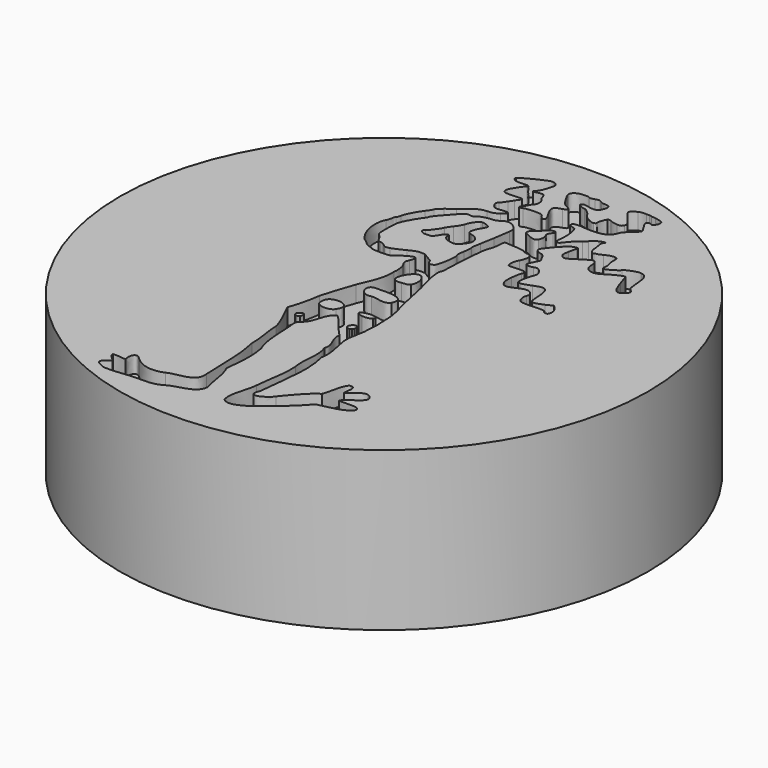
from build123d import *

# Parameters (mm, degrees)
F0_R     = 80
F1_DEPTH = 48
F3_DEPTH = 5


# Not quite as in the source:
# - ends of sketch curves that miss each other by under 0.0002 mm in the source are joined


with BuildPart() as f1:
    # F0 (on Top) → F1 (new body)
    with BuildSketch(Plane.XY):
        Circle(F0_R)
    extrude(amount=F1_DEPTH)

    # F2 (on face) → F3 (cut)
    with BuildSketch(Plane.XY.offset(48)):
        with BuildLine():
            add(Edge.make_bspline(
                [(24.522725, 70.595034), (24.233063, 70.702186), (24.086779, 70.724752), (23.891583, 70.722918)],
                knots=[0, 0, 0, 0, 1, 1, 1, 1], degree=3))
            add(Edge.make_bspline(
                [(23.891583, 70.722918), (23.696395, 70.720937), (23.451897, 70.694859), (22.966103, 70.705838)],
                knots=[0, 0, 0, 0, 1, 1, 1, 1], degree=3))
            add(Edge.make_bspline(
                [(22.966103, 70.705838), (22.184409, 70.723505), (21.250285, 70.779224), (20.571622, 70.377314)],
                knots=[0, 0, 0, 0, 1, 1, 1, 1], degree=3))
            add(Edge.make_bspline(
                [(20.571622, 70.377314), (19.890033, 69.973671), (18.8612, 69.219207), (18.8612, 68.802492)],
                knots=[0, 0, 0, 0, 1, 1, 1, 1], degree=3))
            add(Edge.make_bspline(
                [(18.8612, 68.802492), (18.8612, 68.689275), (19.337049, 68.113525), (19.831339, 67.453667)],
                knots=[0, 0, 0, 0, 1, 1, 1, 1], degree=3))
            add(Edge.make_bspline(
                [(19.831339, 67.453667), (21.496927, 65.230168), (22.01242, 64.899948), (22.413232, 64.067551)],
                knots=[0, 0, 0, 0, 1, 1, 1, 1], degree=3))
            add(Edge.make_bspline(
                [(22.413232, 64.067551), (22.937084, 63.513009), (22.843567, 63.926617), (22.422602, 62.96512)],
                knots=[0, 0, 0, 0, 1, 1, 1, 1], degree=3))
            add(Edge.make_bspline(
                [(22.422602, 62.96512), (22.164591, 62.288128), (21.88761, 62.167018), (20.751869, 62.235863)],
                knots=[0, 0, 0, 0, 1, 1, 1, 1], degree=3))
            add(Edge.make_bspline(
                [(20.751869, 62.235863), (20.002978, 62.281262), (19.029935, 62.508202), (18.589451, 62.740226)],
                knots=[0, 0, 0, 0, 1, 1, 1, 1], degree=3))
            add(Edge.make_bspline(
                [(18.589451, 62.740226), (18.100083, 62.997999), (17.672664, 63.03436), (17.490881, 62.833932)],
                knots=[0, 0, 0, 0, 1, 1, 1, 1], degree=3))
            add(Edge.make_bspline(
                [(17.490881, 62.833932), (17.038191, 62.334819), (16.376702, 60.170166), (16.577517, 59.845244)],
                knots=[0, 0, 0, 0, 1, 1, 1, 1], degree=3))
            add(Edge.make_bspline(
                [(16.577517, 59.845244), (16.675025, 59.687473), (16.42429, 59.453686), (16.020238, 59.325447)],
                knots=[0, 0, 0, 0, 1, 1, 1, 1], degree=3))
            add(Edge.make_bspline(
                [(16.020238, 59.325447), (15.219529, 59.071311), (12.594199, 60.644373), (12.228428, 61.597556)],
                knots=[0, 0, 0, 0, 1, 1, 1, 1], degree=3))
            add(Edge.make_bspline(
                [(12.228428, 61.597556), (11.952922, 62.315509), (10.32579, 63.715941), (9.751267, 63.729657)],
                knots=[0, 0, 0, 0, 1, 1, 1, 1], degree=3))
            add(Edge.make_bspline(
                [(9.751267, 63.729657), (9.494504, 63.735781), (7.426648, 64.17), (7.647828, 64.937921)],
                knots=[0, 0, 0, 0, 1, 1, 1, 1], degree=3))
            add(Edge.make_bspline(
                [(7.647828, 64.937921), (8.277054, 65.725744), (9.846808, 64.956576), (10.980478, 64.886105)],
                knots=[0, 0, 0, 0, 1, 1, 1, 1], degree=3))
            add(Edge.make_bspline(
                [(10.980478, 64.886105), (12.577906, 64.786825), (13.067226, 65.165762), (13.559613, 66.882607)],
                knots=[0, 0, 0, 0, 1, 1, 1, 1], degree=3))
            add(Edge.make_bspline(
                [(13.559613, 66.882607), (13.916173, 68.125864), (13.360638, 68.640806), (11.806198, 68.507592)],
                knots=[0, 0, 0, 0, 1, 1, 1, 1], degree=3))
            add(Edge.make_bspline(
                [(11.806198, 68.507592), (11.321405, 68.466043), (10.853308, 68.801899), (10.525724, 68.977227)],
                knots=[0, 0, 0, 0, 1, 1, 1, 1], degree=3))
            add(Edge.make_bspline(
                [(10.525724, 68.977227), (9.877545, 69.324143), (9.924196, 69.461782), (8.597574, 69.064318)],
                knots=[0, 0, 0, 0, 1, 1, 1, 1], degree=3))
            add(Edge.make_bspline(
                [(8.597574, 69.064318), (7.506288, 68.73736), (7.030529, 68.71743), (6.937864, 68.995416)],
                knots=[0, 0, 0, 0, 1, 1, 1, 1], degree=3))
            add(Edge.make_bspline(
                [(6.937864, 68.995416), (6.866423, 69.209738), (5.719491, 69.108415), (4.974436, 69.108415)],
                knots=[0, 0, 0, 0, 1, 1, 1, 1], degree=3))
            add(Edge.make_bspline(
                [(4.974436, 69.108415), (3.344859, 69.108415), (1.845701, 67.945318), (2.159379, 66.98734)],
                knots=[0, 0, 0, 0, 1, 1, 1, 1], degree=3))
            add(Edge.make_bspline(
                [(2.159379, 66.98734), (2.644291, 65.506427), (3.555651, 64.36065), (3.708294, 64.093459)],
                knots=[0, 0, 0, 0, 1, 1, 1, 1], degree=3))
            Line((3.708294, 64.093459), (4.061072, 63.476097))
            add(Edge.make_bspline(
                [(4.061072, 63.476097), (4.241169, 63.16085), (4.670435, 62.567618), (5.51683, 62.152077)],
                knots=[0, 0, 0, 0, 1, 1, 1, 1], degree=3))
            add(Edge.make_bspline(
                [(5.51683, 62.152077), (7.271411, 61.290653), (7.334279, 60.85184), (5.768186, 60.389292)],
                knots=[0, 0, 0, 0, 1, 1, 1, 1], degree=3))
            add(Edge.make_bspline(
                [(5.768186, 60.389292), (3.30002, 59.660317), (3.118873, 58.929393), (4.750089, 56.278327)],
                knots=[0, 0, 0, 0, 1, 1, 1, 1], degree=3))
            add(Edge.make_bspline(
                [(4.750089, 56.278327), (5.332172, 55.332321), (5.808422, 54.322457), (5.808422, 54.03433)],
                knots=[0, 0, 0, 0, 1, 1, 1, 1], degree=3))
            add(Edge.make_bspline(
                [(5.808422, 54.03433), (5.808422, 53.210239), (4.889352, 53.42155), (4.253446, 54.39207)],
                knots=[0, 0, 0, 0, 1, 1, 1, 1], degree=3))
            add(Edge.make_bspline(
                [(4.253446, 54.39207), (3.73622, 55.181454), (3.437231, 55.274014), (1.406969, 55.274014)],
                knots=[0, 0, 0, 0, 1, 1, 1, 1], degree=3))
            add(Edge.make_bspline(
                [(1.406969, 55.274014), (0.159392, 55.274014), (-1.266395, 55.089458), (-1.761416, 54.863911)],
                knots=[0, 0, 0, 0, 1, 1, 1, 1], degree=3))
            add(Edge.make_bspline(
                [(-1.761416, 54.863911), (-2.993516, 54.302529), (-3.294449, 54.750966), (-2.356176, 55.749714)],
                knots=[0, 0, 0, 0, 1, 1, 1, 1], degree=3))
            add(Edge.make_bspline(
                [(-2.356176, 55.749714), (-1.929724, 56.203648), (-1.687482, 57.017572), (-1.423522, 57.390681)],
                knots=[0, 0, 0, 0, 1, 1, 1, 1], degree=3))
            add(Edge.make_bspline(
                [(-1.423522, 57.390681), (-1.03471, 57.940266), (-0.466679, 58.411795), (-0.481495, 59.042121)],
                knots=[0, 0, 0, 0, 1, 1, 1, 1], degree=3))
            Line((-0.481495, 59.042121), (-1.001298, 60.953186))
            add(Edge.make_bspline(
                [(-1.001298, 60.953186), (-1.99067, 61.768707), (-1.593124, 62.769955), (-2.273976, 63.235297)],
                knots=[0, 0, 0, 0, 1, 1, 1, 1], degree=3))
            add(Edge.make_bspline(
                [(-2.273976, 63.235297), (-3.104235, 63.80275), (-5.087721, 62.734017), (-5.282036, 62.999297)],
                knots=[0, 0, 0, 0, 1, 1, 1, 1], degree=3))
            add(Edge.make_bspline(
                [(-5.282036, 62.999297), (-5.39946, 63.189292), (-5.293607, 63.473543), (-5.046668, 63.630989)],
                knots=[0, 0, 0, 0, 1, 1, 1, 1], degree=3))
            add(Edge.make_bspline(
                [(-5.046668, 63.630989), (-4.481129, 63.991582), (-3.871625, 65.249317), (-3.319711, 67.195699)],
                knots=[0, 0, 0, 0, 1, 1, 1, 1], degree=3))
            add(Edge.make_bspline(
                [(-3.319711, 67.195699), (-2.952041, 68.492326), (-2.970916, 68.790489), (-3.448695, 69.268268)],
                knots=[0, 0, 0, 0, 1, 1, 1, 1], degree=3))
            add(Edge.make_bspline(
                [(-3.448695, 69.268268), (-3.755629, 69.575205), (-4.378445, 69.826097), (-4.832795, 69.826097)],
                knots=[0, 0, 0, 0, 1, 1, 1, 1], degree=3))
            add(Edge.make_bspline(
                [(-4.832795, 69.826097), (-5.867523, 69.826097), (-12.562215, 66.553353), (-12.801164, 65.93066)],
                knots=[0, 0, 0, 0, 1, 1, 1, 1], degree=3))
            add(Edge.make_bspline(
                [(-12.801164, 65.93066), (-13.103503, 65.142783), (-11.77094, 64.413888), (-10.33117, 64.579631)],
                knots=[0, 0, 0, 0, 1, 1, 1, 1], degree=3))
            add(Edge.make_bspline(
                [(-10.33117, 64.579631), (-9.158629, 64.71461), (-7.35364, 64.903716), (-8.086619, 64.186614)],
                knots=[0, 0, 0, 0, 1, 1, 1, 1], degree=3))
            add(Edge.make_bspline(
                [(-8.086619, 64.186614), (-8.451558, 63.829584), (-10.772142, 60.580706), (-10.772142, 59.695313)],
                knots=[0, 0, 0, 0, 1, 1, 1, 1], degree=3))
            add(Edge.make_bspline(
                [(-10.772142, 59.695313), (-10.772142, 58.627779), (-10.244513, 58.293024), (-8.72217, 58.395547)],
                knots=[0, 0, 0, 0, 1, 1, 1, 1], degree=3))
            add(Edge.make_bspline(
                [(-8.72217, 58.395547), (-7.82656, 58.455864), (-6.579872, 58.530695), (-5.651349, 58.549886)],
                knots=[0, 0, 0, 0, 1, 1, 1, 1], degree=3))
            add(Edge.make_bspline(
                [(-5.651349, 58.549886), (-3.885942, 58.586366), (-5.648809, 57.191723), (-5.842072, 56.658117)],
                knots=[0, 0, 0, 0, 1, 1, 1, 1], degree=3))
            Line((-5.842072, 56.658117), (-6.67165, 55.343466))
            add(Edge.make_bspline(
                [(-6.67165, 55.343466), (-7.128023, 54.620523), (-7.751509, 53.821326), (-8.057407, 53.567453)],
                knots=[0, 0, 0, 0, 1, 1, 1, 1], degree=3))
            add(Edge.make_bspline(
                [(-8.057407, 53.567453), (-8.656912, 53.069906), (-8.521332, 52.301858), (-7.656121, 51.295341)],
                knots=[0, 0, 0, 0, 1, 1, 1, 1], degree=3))
            add(Edge.make_bspline(
                [(-7.656121, 51.295341), (-7.204923, 50.77045), (-6.780399, 50.705353), (-5.063754, 50.89957)],
                knots=[0, 0, 0, 0, 1, 1, 1, 1], degree=3))
            add(Edge.make_bspline(
                [(-5.063754, 50.89957), (-2.627062, 51.17525), (-2.439217, 50.807322), (-4.294809, 49.391995)],
                knots=[0, 0, 0, 0, 1, 1, 1, 1], degree=3))
            add(Edge.make_bspline(
                [(-4.294809, 49.391995), (-5.284181, 48.637364), (-6.002764, 48.400218), (-7.426265, 48.359019)],
                knots=[0, 0, 0, 0, 1, 1, 1, 1], degree=3))
            add(Edge.make_bspline(
                [(-7.426265, 48.359019), (-9.266164, 48.305767), (-10.477911, 47.639505), (-13.85674, 44.821869)],
                knots=[0, 0, 0, 0, 1, 1, 1, 1], degree=3))
            add(Edge.make_bspline(
                [(-13.85674, 44.821869), (-14.29202, 44.458883), (-15.363584, 43.606643), (-16.23799, 42.928446)],
                knots=[0, 0, 0, 0, 1, 1, 1, 1], degree=3))
            add(Edge.make_bspline(
                [(-16.23799, 42.928446), (-17.112397, 42.250252), (-17.827697, 41.518997), (-17.827697, 41.303464)],
                knots=[0, 0, 0, 0, 1, 1, 1, 1], degree=3))
            add(Edge.make_bspline(
                [(-17.827697, 41.303464), (-17.827697, 41.087928), (-18.359957, 40.214052), (-19.010604, 39.361532)],
                knots=[0, 0, 0, 0, 1, 1, 1, 1], degree=3))
            add(Edge.make_bspline(
                [(-19.010604, 39.361532), (-20.451382, 37.473734), (-21.538646, 35.376204), (-21.868657, 33.847175)],
                knots=[0, 0, 0, 0, 1, 1, 1, 1], degree=3))
            add(Edge.make_bspline(
                [(-21.868657, 33.847175), (-22.004279, 33.218807), (-22.262266, 32.614005), (-22.441367, 32.503312)],
                knots=[0, 0, 0, 0, 1, 1, 1, 1], degree=3))
            add(Edge.make_bspline(
                [(-22.441367, 32.503312), (-22.620468, 32.392622), (-22.766586, 31.986114), (-22.766586, 31.599871)],
                knots=[0, 0, 0, 0, 1, 1, 1, 1], degree=3))
            add(Edge.make_bspline(
                [(-22.766586, 31.599871), (-22.766586, 31.21363), (-23.001545, 30.443423), (-23.288587, 29.888345)],
                knots=[0, 0, 0, 0, 1, 1, 1, 1], degree=3))
            add(Edge.make_bspline(
                [(-23.288587, 29.888345), (-24.543423, 27.461756), (-24.119368, 23.492182), (-22.297502, 20.613597)],
                knots=[0, 0, 0, 0, 1, 1, 1, 1], degree=3))
            add(Edge.make_bspline(
                [(-22.297502, 20.613597), (-21.714196, 19.691967), (-21.13351, 18.937903), (-21.007106, 18.937903)],
                knots=[0, 0, 0, 0, 1, 1, 1, 1], degree=3))
            add(Edge.make_bspline(
                [(-21.007106, 18.937903), (-20.880701, 18.937903), (-20.243562, 18.461653), (-19.591586, 17.87957)],
                knots=[0, 0, 0, 0, 1, 1, 1, 1], degree=3))
            add(Edge.make_bspline(
                [(-19.591586, 17.87957), (-18.939611, 17.297486), (-18.126912, 16.821236), (-17.785254, 16.821236)],
                knots=[0, 0, 0, 0, 1, 1, 1, 1], degree=3))
            add(Edge.make_bspline(
                [(-17.785254, 16.821236), (-17.443596, 16.821236), (-17.065669, 16.662486), (-16.945753, 16.468459)],
                knots=[0, 0, 0, 0, 1, 1, 1, 1], degree=3))
            add(Edge.make_bspline(
                [(-16.945753, 16.468459), (-16.648025, 15.986728), (-11.229864, 16.013584), (-10.930339, 16.498224)],
                knots=[0, 0, 0, 0, 1, 1, 1, 1], degree=3))
            add(Edge.make_bspline(
                [(-10.930339, 16.498224), (-10.800474, 16.708353), (-9.846244, 17.422728), (-8.809814, 18.085724)],
                knots=[0, 0, 0, 0, 1, 1, 1, 1], degree=3))
            add(Edge.make_bspline(
                [(-8.809814, 18.085724), (-5.96062, 19.90833), (-5.06882, 19.657067), (-6.049878, 17.309063)],
                knots=[0, 0, 0, 0, 1, 1, 1, 1], degree=3))
            add(Edge.make_bspline(
                [(-6.049878, 17.309063), (-6.574586, 16.053267), (-6.570516, 15.87637), (-5.992003, 14.802134)],
                knots=[0, 0, 0, 0, 1, 1, 1, 1], degree=3))
            Line((-5.992003, 14.802134), (-5.388973, 13.682618))
            add(Edge.make_bspline(
                [(-5.388973, 13.682618), (-5.278994, 12.380882), (-4.98303, 11.387617), (-5.299125, 10.435408)],
                knots=[0, 0, 0, 0, 1, 1, 1, 1], degree=3))
            add(Edge.make_bspline(
                [(-5.299125, 10.435408), (-4.924624, 6.564533), (-6.784054, 3.047559), (-8.216707, -0.421328)],
                knots=[0, 0, 0, 0, 1, 1, 1, 1], degree=3))
            add(Edge.make_bspline(
                [(-8.216707, -0.421328), (-9.516716, -3.60075), (-10.262812, -7.024907), (-11.352018, -10.214769)],
                knots=[0, 0, 0, 0, 1, 1, 1, 1], degree=3))
            add(Edge.make_bspline(
                [(-11.352018, -10.214769), (-11.76474, -13.396102), (-12.493974, -16.532977), (-13.600976, -19.556215)],
                knots=[0, 0, 0, 0, 1, 1, 1, 1], degree=3))
            add(Edge.make_bspline(
                [(-13.600976, -19.556215), (-12.288014, -22.651919), (-10.395127, -25.54803), (-9.642149, -28.840886)],
                knots=[0, 0, 0, 0, 1, 1, 1, 1], degree=3))
            add(Edge.make_bspline(
                [(-9.642149, -28.840886), (-9.594586, -32.330778), (-8.556401, -35.691054), (-8.657129, -39.19326)],
                knots=[0, 0, 0, 0, 1, 1, 1, 1], degree=3))
            add(Edge.make_bspline(
                [(-8.657129, -39.19326), (-7.144872, -45.432631), (-7.605439, -51.929971), (-7.175462, -58.301688)],
                knots=[0, 0, 0, 0, 1, 1, 1, 1], degree=3))
            add(Edge.make_bspline(
                [(-7.175462, -58.301688), (-6.548257, -63.167792), (-12.406347, -62.239501), (-15.176902, -63.733365)],
                knots=[0, 0, 0, 0, 1, 1, 1, 1], degree=3))
            add(Edge.make_bspline(
                [(-15.176902, -63.733365), (-18.35449, -65.081752), (-21.9356, -64.681172), (-24.805532, -61.775448)],
                knots=[0, 0, 0, 0, 1, 1, 1, 1], degree=3))
            add(Edge.make_bspline(
                [(-24.805532, -61.775448), (-26.688817, -59.868676), (-27.554608, -62.666003), (-26.80975, -64.276313)],
                knots=[0, 0, 0, 0, 1, 1, 1, 1], degree=3))
            add(Edge.make_bspline(
                [(-26.80975, -64.276313), (-27.921759, -64.34338), (-29.646639, -63.821187), (-30.850709, -64.100474)],
                knots=[0, 0, 0, 0, 1, 1, 1, 1], degree=3))
            add(Edge.make_bspline(
                [(-30.850709, -64.100474), (-30.948059, -65.198186), (-29.302621, -65.920497), (-28.85531, -66.779381)],
                knots=[0, 0, 0, 0, 1, 1, 1, 1], degree=3))
            add(Edge.make_bspline(
                [(-28.85531, -66.779381), (-29.513899, -67.358645), (-31.134712, -68.204657), (-31.027648, -68.991958)],
                knots=[0, 0, 0, 0, 1, 1, 1, 1], degree=3))
            add(Edge.make_bspline(
                [(-31.027648, -68.991958), (-30.9415, -69.625482), (-29.687355, -70.078505), (-28.880115, -70.481894)],
                knots=[0, 0, 0, 0, 1, 1, 1, 1], degree=3))
            add(Edge.make_bspline(
                [(-28.880115, -70.481894), (-27.886806, -70.978264), (-24.254227, -70.618213), (-20.843947, -70.234396)],
                knots=[0, 0, 0, 0, 1, 1, 1, 1], degree=3))
            add(Edge.make_bspline(
                [(-20.843947, -70.234396), (-17.203879, -69.82472), (-14.587414, -70.820267), (-11.188309, -68.767061)],
                knots=[0, 0, 0, 0, 1, 1, 1, 1], degree=3))
            add(Edge.make_bspline(
                [(-11.188309, -68.767061), (-8.339423, -67.046211), (-3.293405, -67.463691), (-2.78448, -63.458859)],
                knots=[0, 0, 0, 0, 1, 1, 1, 1], degree=3))
            add(Edge.make_bspline(
                [(-2.78448, -63.458859), (-3.80083, -60.019916), (-3.686905, -56.22129), (-5.34653, -52.992936)],
                knots=[0, 0, 0, 0, 1, 1, 1, 1], degree=3))
            add(Edge.make_bspline(
                [(-5.34653, -52.992936), (-4.769221, -48.662913), (-4.445165, -44.226047), (-5.272116, -39.898265)],
                knots=[0, 0, 0, 0, 1, 1, 1, 1], degree=3))
            add(Edge.make_bspline(
                [(-5.272116, -39.898265), (-7.076828, -35.924105), (-6.637115, -31.423476), (-7.08396, -27.18283)],
                knots=[0, 0, 0, 0, 1, 1, 1, 1], degree=3))
            add(Edge.make_bspline(
                [(-7.08396, -27.18283), (-7.080348, -25.874589), (-7.812994, -24.338671), (-6.495812, -23.43677)],
                knots=[0, 0, 0, 0, 1, 1, 1, 1], degree=3))
            add(Edge.make_bspline(
                [(-6.495812, -23.43677), (-3.657511, -21.438298), (-4.723445, -17.065558), (-1.698034, -15.503131)],
                knots=[0, 0, 0, 0, 1, 1, 1, 1], degree=3))
            add(Edge.make_bspline(
                [(-1.698034, -15.503131), (0.752634, -17.577222), (2.513396, -20.758016), (4.987655, -23.098324)],
                knots=[0, 0, 0, 0, 1, 1, 1, 1], degree=3))
            add(Edge.make_bspline(
                [(4.987655, -23.098324), (4.468572, -25.888734), (7.265903, -27.84126), (6.248836, -30.426181)],
                knots=[0, 0, 0, 0, 1, 1, 1, 1], degree=3))
            add(Edge.make_bspline(
                [(6.248836, -30.426181), (7.792834, -34.182745), (6.084712, -38.118975), (6.863993, -42.052413)],
                knots=[0, 0, 0, 0, 1, 1, 1, 1], degree=3))
            add(Edge.make_bspline(
                [(6.863993, -42.052413), (7.267404, -46.592401), (5.98027, -50.972433), (5.675021, -55.459623)],
                knots=[0, 0, 0, 0, 1, 1, 1, 1], degree=3))
            add(Edge.make_bspline(
                [(5.675021, -55.459623), (5.45009, -58.853489), (3.239842, -62.464308), (4.27383, -65.71829)],
                knots=[0, 0, 0, 0, 1, 1, 1, 1], degree=3))
            add(Edge.make_bspline(
                [(4.27383, -65.71829), (6.321254, -67.698903), (9.067304, -65.697152), (11.100634, -64.674288)],
                knots=[0, 0, 0, 0, 1, 1, 1, 1], degree=3))
            add(Edge.make_bspline(
                [(11.100634, -64.674288), (14.302829, -62.398968), (20.279166, -57.238122), (22.590716, -54.275613)],
                knots=[0, 0, 0, 0, 1, 1, 1, 1], degree=3))
            add(Edge.make_bspline(
                [(22.590716, -54.275613), (29.35799, -52.498403), (26.515086, -53.637283), (29.357984, -52.498494)],
                knots=[0, 0, 0, 0, 1, 1, 1, 1], degree=3))
            add(Edge.make_bspline(
                [(29.357984, -52.498494), (31.767933, -51.533133), (32.611854, -50.238955), (31.417876, -49.594142)],
                knots=[0, 0, 0, 0, 1, 1, 1, 1], degree=3))
            add(Edge.make_bspline(
                [(31.417876, -49.594142), (30.252369, -48.964704), (27.262572, -49.627252), (25.780047, -49.225379)],
                knots=[0, 0, 0, 0, 1, 1, 1, 1], degree=3))
            add(Edge.make_bspline(
                [(25.780047, -49.225379), (27.399413, -46.878346), (32.183263, -45.657675), (30.386001, -43.392419)],
                knots=[0, 0, 0, 0, 1, 1, 1, 1], degree=3))
            add(Edge.make_bspline(
                [(30.386001, -43.392419), (28.576624, -41.111891), (25.640124, -44.473697), (24.21239, -45.430811)],
                knots=[0, 0, 0, 0, 1, 1, 1, 1], degree=3))
            add(Edge.make_bspline(
                [(24.21239, -45.430811), (24.106323, -44.2573), (25.213703, -41.723009), (23.404859, -41.664358)],
                knots=[0, 0, 0, 0, 1, 1, 1, 1], degree=3))
            add(Edge.make_bspline(
                [(23.404859, -41.664358), (21.655973, -41.607651), (21.36426, -47.486179), (20.491688, -49.066076)],
                knots=[0, 0, 0, 0, 1, 1, 1, 1], degree=3))
            add(Edge.make_bspline(
                [(20.491688, -49.066076), (17.432701, -51.023665), (15.187742, -54.106751), (12.836961, -56.890027)],
                knots=[0, 0, 0, 0, 1, 1, 1, 1], degree=3))
            add(Edge.make_bspline(
                [(12.836961, -56.890027), (11.70214, -58.882414), (6.153837, -61.653105), (8.193525, -57.148548)],
                knots=[0, 0, 0, 0, 1, 1, 1, 1], degree=3))
            add(Edge.make_bspline(
                [(8.193525, -57.148548), (8.861993, -52.678819), (9.028414, -48.153256), (9.525811, -43.663617)],
                knots=[0, 0, 0, 0, 1, 1, 1, 1], degree=3))
            add(Edge.make_bspline(
                [(9.525811, -43.663617), (9.752074, -40.723739), (9.420867, -37.419326), (8.7271, -34.521711)],
                knots=[0, 0, 0, 0, 1, 1, 1, 1], degree=3))
            add(Edge.make_bspline(
                [(8.7271, -34.521711), (9.575747, -30.47423), (7.287817, -26.702595), (7.642858, -22.693182)],
                knots=[0, 0, 0, 0, 1, 1, 1, 1], degree=3))
            add(Edge.make_bspline(
                [(7.642858, -22.693182), (8.740491, -18.063412), (8.900751, -13.274402), (8.485667, -8.540729)],
                knots=[0, 0, 0, 0, 1, 1, 1, 1], degree=3))
            add(Edge.make_bspline(
                [(8.485667, -8.540729), (8.260499, -4.973321), (6.723406, -1.712308), (6.232851, 1.721244)],
                knots=[0, 0, 0, 0, 1, 1, 1, 1], degree=3))
            add(Edge.make_bspline(
                [(6.232851, 1.721244), (5.362816, 5.562302), (4.627458, 9.90049), (3.427164, 13.667733)],
                knots=[0, 0, 0, 0, 1, 1, 1, 1], degree=3))
            Line((3.427164, 13.667733), (3.198962, 15.384217))
            add(Edge.make_bspline(
                [(3.198962, 15.384217), (3.069015, 16.363805), (3.113561, 17.211451), (3.300937, 17.327252)],
                knots=[0, 0, 0, 0, 1, 1, 1, 1], degree=3))
            add(Edge.make_bspline(
                [(3.300937, 17.327252), (3.483747, 17.440237), (3.624779, 18.682608), (3.614026, 20.087738)],
                knots=[0, 0, 0, 0, 1, 1, 1, 1], degree=3))
            add(Edge.make_bspline(
                [(3.614026, 20.087738), (3.603273, 21.492872), (3.713052, 23.832695), (3.858216, 25.287903)],
                knots=[0, 0, 0, 0, 1, 1, 1, 1], degree=3))
            add(Edge.make_bspline(
                [(3.858216, 25.287903), (4.00338, 26.743111), (4.171017, 28.648111), (4.230837, 29.521236)],
                knots=[0, 0, 0, 0, 1, 1, 1, 1], degree=3))
            add(Edge.make_bspline(
                [(4.230837, 29.521236), (4.379094, 31.685215), (4.619705, 32.941304), (5.113885, 34.134356)],
                knots=[0, 0, 0, 0, 1, 1, 1, 1], degree=3))
            add(Edge.make_bspline(
                [(5.113885, 34.134356), (5.343478, 34.688649), (5.553629, 35.901578), (5.581315, 36.829798)],
                knots=[0, 0, 0, 0, 1, 1, 1, 1], degree=3))
            add(Edge.make_bspline(
                [(5.581315, 36.829798), (5.628342, 38.405787), (5.690391, 38.51149), (6.513969, 38.432733)],
                knots=[0, 0, 0, 0, 1, 1, 1, 1], degree=3))
            add(Edge.make_bspline(
                [(6.513969, 38.432733), (6.999039, 38.386347), (8.389627, 38.29806), (9.604083, 38.235951)],
                knots=[0, 0, 0, 0, 1, 1, 1, 1], degree=3))
            add(Edge.make_bspline(
                [(9.604083, 38.235951), (10.818533, 38.173842), (12.001222, 37.933979), (12.232277, 37.702926)],
                knots=[0, 0, 0, 0, 1, 1, 1, 1], degree=3))
            add(Edge.make_bspline(
                [(12.232277, 37.702926), (12.463327, 37.471874), (13.079531, 37.282347), (13.602048, 37.282347)],
                knots=[0, 0, 0, 0, 1, 1, 1, 1], degree=3))
            add(Edge.make_bspline(
                [(13.602048, 37.282347), (15.144847, 37.282347), (15.426578, 35.658912), (14.27508, 33.401792)],
                knots=[0, 0, 0, 0, 1, 1, 1, 1], degree=3))
            add(Edge.make_bspline(
                [(14.27508, 33.401792), (13.480334, 31.843965), (13.346372, 30.010452), (14.010497, 29.780308)],
                knots=[0, 0, 0, 0, 1, 1, 1, 1], degree=3))
            add(Edge.make_bspline(
                [(14.010497, 29.780308), (14.253033, 29.696254), (15.421701, 29.70288), (16.607825, 29.795181)],
                knots=[0, 0, 0, 0, 1, 1, 1, 1], degree=3))
            add(Edge.make_bspline(
                [(16.607825, 29.795181), (18.934355, 29.976246), (19.499048, 29.65591), (18.882691, 28.504234)],
                knots=[0, 0, 0, 0, 1, 1, 1, 1], degree=3))
            add(Edge.make_bspline(
                [(18.882691, 28.504234), (18.682765, 28.130671), (18.417386, 26.724276), (18.292339, 25.378846)],
                knots=[0, 0, 0, 0, 1, 1, 1, 1], degree=3))
            add(Edge.make_bspline(
                [(18.292339, 25.378846), (18.106614, 23.380498), (18.17735, 22.760733), (18.679844, 21.993833)],
                knots=[0, 0, 0, 0, 1, 1, 1, 1], degree=3))
            add(Edge.make_bspline(
                [(18.679844, 21.993833), (19.447793, 20.821804), (20.164288, 20.816182), (22.590716, 21.964067)],
                knots=[0, 0, 0, 0, 1, 1, 1, 1], degree=3))
            add(Edge.make_bspline(
                [(22.590716, 21.964067), (23.997089, 22.629367), (24.801772, 22.80989), (25.590981, 22.636549)],
                knots=[0, 0, 0, 0, 1, 1, 1, 1], degree=3))
            add(Edge.make_bspline(
                [(25.590981, 22.636549), (26.760716, 22.379637), (27.434123, 21.241728), (26.956891, 20.328612)],
                knots=[0, 0, 0, 0, 1, 1, 1, 1], degree=3))
            add(Edge.make_bspline(
                [(26.956891, 20.328612), (26.508209, 19.470123), (26.824927, 17.803401), (27.535667, 17.283697)],
                knots=[0, 0, 0, 0, 1, 1, 1, 1], degree=3))
            add(Edge.make_bspline(
                [(27.535667, 17.283697), (28.013681, 16.934159), (29.060954, 16.860626), (31.594816, 16.998167)],
                knots=[0, 0, 0, 0, 1, 1, 1, 1], degree=3))
            add(Edge.make_bspline(
                [(31.594816, 16.998167), (34.435278, 17.152354), (35.044274, 17.09379), (35.214649, 16.6498)],
                knots=[0, 0, 0, 0, 1, 1, 1, 1], degree=3))
            add(Edge.make_bspline(
                [(35.214649, 16.6498), (35.327306, 16.356222), (35.74213, 16.115672), (36.136279, 16.115672)],
                knots=[0, 0, 0, 0, 1, 1, 1, 1], degree=3))
            add(Edge.make_bspline(
                [(36.136279, 16.115672), (37.246567, 16.115672), (37.141766, 18.543212), (35.984695, 19.630222)],
                knots=[0, 0, 0, 0, 1, 1, 1, 1], degree=3))
            Line((35.984695, 19.630222), (33.215389, 19.51557))
            add(Edge.make_bspline(
                [(33.215389, 19.51557), (31.181261, 18.520364), (29.988206, 18.34358), (29.595009, 18.979788)],
                knots=[0, 0, 0, 0, 1, 1, 1, 1], degree=3))
            add(Edge.make_bspline(
                [(29.595009, 18.979788), (29.460837, 19.196876), (29.312281, 20.347812), (29.264828, 21.537426)],
                knots=[0, 0, 0, 0, 1, 1, 1, 1], degree=3))
            add(Edge.make_bspline(
                [(29.264828, 21.537426), (29.087788, 25.975605), (28.18101, 26.739282), (24.787858, 25.307738)],
                knots=[0, 0, 0, 0, 1, 1, 1, 1], degree=3))
            add(Edge.make_bspline(
                [(24.787858, 25.307738), (23.504075, 24.766119), (22.085027, 24.34175), (21.634358, 24.36461)],
                knots=[0, 0, 0, 0, 1, 1, 1, 1], degree=3))
            add(Edge.make_bspline(
                [(21.634358, 24.36461), (20.88639, 24.402569), (20.825142, 24.544346), (20.929353, 25.99345)],
                knots=[0, 0, 0, 0, 1, 1, 1, 1], degree=3))
            add(Edge.make_bspline(
                [(20.929353, 25.99345), (20.992144, 26.866575), (21.266538, 28.116743), (21.539548, 28.771025)],
                knots=[0, 0, 0, 0, 1, 1, 1, 1], degree=3))
            add(Edge.make_bspline(
                [(21.539548, 28.771025), (22.238982, 30.447241), (22.163621, 31.111671), (21.148735, 32.20675)],
                knots=[0, 0, 0, 0, 1, 1, 1, 1], degree=3))
            add(Edge.make_bspline(
                [(21.148735, 32.20675), (20.331346, 33.088731), (20.161471, 33.133692), (19.000099, 32.777257)],
                knots=[0, 0, 0, 0, 1, 1, 1, 1], degree=3))
            add(Edge.make_bspline(
                [(19.000099, 32.777257), (17.725693, 32.386128), (16.744525, 32.516867), (16.744525, 33.077668)],
                knots=[0, 0, 0, 0, 1, 1, 1, 1], degree=3))
            add(Edge.make_bspline(
                [(16.744525, 33.077668), (16.744525, 33.245746), (17.085774, 34.085867), (17.502997, 34.944636)],
                knots=[0, 0, 0, 0, 1, 1, 1, 1], degree=3))
            Line((17.502997, 34.944636), (17.558671, 37.864422))
            add(Edge.make_bspline(
                [(17.558671, 37.864422), (17.090831, 38.768645), (16.57189, 39.263782), (16.006449, 39.344985)],
                knots=[0, 0, 0, 0, 1, 1, 1, 1], degree=3))
            add(Edge.make_bspline(
                [(16.006449, 39.344985), (14.960378, 39.495218), (14.27508, 40.028663), (14.27508, 40.692707)],
                knots=[0, 0, 0, 0, 1, 1, 1, 1], degree=3))
            add(Edge.make_bspline(
                [(14.27508, 40.692707), (14.27508, 41.403591), (17.678599, 45.413347), (19.115302, 46.395029)],
                knots=[0, 0, 0, 0, 1, 1, 1, 1], degree=3))
            add(Edge.make_bspline(
                [(19.115302, 46.395029), (20.24228, 47.165084), (21.627387, 47.220969), (21.168028, 46.477712)],
                knots=[0, 0, 0, 0, 1, 1, 1, 1], degree=3))
            add(Edge.make_bspline(
                [(21.168028, 46.477712), (21.054205, 46.293542), (20.795345, 45.245228), (20.59256, 44.148278)],
                knots=[0, 0, 0, 0, 1, 1, 1, 1], degree=3))
            add(Edge.make_bspline(
                [(20.59256, 44.148278), (20.272794, 42.418481), (20.304993, 42.064058), (20.836197, 41.477087)],
                knots=[0, 0, 0, 0, 1, 1, 1, 1], degree=3))
            add(Edge.make_bspline(
                [(20.836197, 41.477087), (21.599439, 40.633711), (22.077484, 40.780317), (25.040868, 42.767483)],
                knots=[0, 0, 0, 0, 1, 1, 1, 1], degree=3))
            add(Edge.make_bspline(
                [(25.040868, 42.767483), (26.328995, 43.631264), (27.576981, 44.337894), (27.814031, 44.337894)],
                knots=[0, 0, 0, 0, 1, 1, 1, 1], degree=3))
            add(Edge.make_bspline(
                [(27.814031, 44.337894), (28.604965, 44.337894), (29.091747, 43.504653), (29.091747, 42.150672)],
                knots=[0, 0, 0, 0, 1, 1, 1, 1], degree=3))
            add(Edge.make_bspline(
                [(29.091747, 42.150672), (29.091747, 39.526443), (31.565665, 38.563123), (34.036701, 40.225279)],
                knots=[0, 0, 0, 0, 1, 1, 1, 1], degree=3))
            add(Edge.make_bspline(
                [(34.036701, 40.225279), (36.349952, 41.7813), (38.986148, 42.945054), (39.142056, 42.478646)],
                knots=[0, 0, 0, 0, 1, 1, 1, 1], degree=3))
            add(Edge.make_bspline(
                [(39.142056, 42.478646), (39.221741, 42.240261), (39.703853, 40.774839), (40.213067, 39.222617)],
                knots=[0, 0, 0, 0, 1, 1, 1, 1], degree=3))
            add(Edge.make_bspline(
                [(40.213067, 39.222617), (41.539234, 35.180122), (42.444541, 34.409452), (44.172997, 35.851385)],
                knots=[0, 0, 0, 0, 1, 1, 1, 1], degree=3))
            add(Edge.make_bspline(
                [(44.172997, 35.851385), (45.153917, 36.669699), (45.183705, 37.399893), (44.262295, 38.033095)],
                knots=[0, 0, 0, 0, 1, 1, 1, 1], degree=3))
            add(Edge.make_bspline(
                [(44.262295, 38.033095), (43.684741, 38.42999), (43.516751, 39.07377), (43.327984, 41.610482)],
                knots=[0, 0, 0, 0, 1, 1, 1, 1], degree=3))
            add(Edge.make_bspline(
                [(43.327984, 41.610482), (43.069728, 45.080977), (42.507982, 46.110913), (40.763733, 46.314)],
                knots=[0, 0, 0, 0, 1, 1, 1, 1], degree=3))
            add(Edge.make_bspline(
                [(40.763733, 46.314), (39.712946, 46.436347), (36.717598, 45.32874), (36.30826, 44.666418)],
                knots=[0, 0, 0, 0, 1, 1, 1, 1], degree=3))
            add(Edge.make_bspline(
                [(36.30826, 44.666418), (35.980515, 44.136117), (33.524197, 42.645176), (32.760086, 42.51282)],
                knots=[0, 0, 0, 0, 1, 1, 1, 1], degree=3))
            add(Edge.make_bspline(
                [(32.760086, 42.51282), (32.205734, 42.416822), (32.113896, 42.586254), (32.206665, 43.536429)],
                knots=[0, 0, 0, 0, 1, 1, 1, 1], degree=3))
            add(Edge.make_bspline(
                [(32.206665, 43.536429), (32.267805, 44.162632), (32.187192, 44.877007), (32.027521, 45.123929)],
                knots=[0, 0, 0, 0, 1, 1, 1, 1], degree=3))
            add(Edge.make_bspline(
                [(32.027521, 45.123929), (31.86784, 45.37085), (31.73758, 46.286992), (31.73758, 47.160117)],
                knots=[0, 0, 0, 0, 1, 1, 1, 1], degree=3))
            add(Edge.make_bspline(
                [(31.73758, 47.160117), (31.73758, 48.638267), (31.66906, 48.755818), (30.745394, 48.861719)],
                knots=[0, 0, 0, 0, 1, 1, 1, 1], degree=3))
            add(Edge.make_bspline(
                [(30.745394, 48.861719), (30.170496, 48.927635), (29.020932, 48.59255), (28.011367, 48.064662)],
                knots=[0, 0, 0, 0, 1, 1, 1, 1], degree=3))
            add(Edge.make_bspline(
                [(28.011367, 48.064662), (27.05325, 47.563678), (26.269525, 47.254105), (26.269525, 47.376745)],
                knots=[0, 0, 0, 0, 1, 1, 1, 1], degree=3))
            add(Edge.make_bspline(
                [(26.269525, 47.376745), (26.269525, 47.499382), (26.061716, 47.427322), (25.808159, 47.216891)],
                knots=[0, 0, 0, 0, 1, 1, 1, 1], degree=3))
            add(Edge.make_bspline(
                [(25.808159, 47.216891), (25.456959, 46.925418), (25.207176, 47.071482), (24.759196, 47.829844)],
                knots=[0, 0, 0, 0, 1, 1, 1, 1], degree=3))
            add(Edge.make_bspline(
                [(24.759196, 47.829844), (24.43578, 48.377347), (24.252113, 48.90585), (24.350747, 49.004484)],
                knots=[0, 0, 0, 0, 1, 1, 1, 1], degree=3))
            add(Edge.make_bspline(
                [(24.350747, 49.004484), (24.449381, 49.103115), (24.374962, 49.874409), (24.185382, 50.718211)],
                knots=[0, 0, 0, 0, 1, 1, 1, 1], degree=3))
            add(Edge.make_bspline(
                [(24.185382, 50.718211), (23.946701, 51.780523), (23.958396, 52.394278), (24.223414, 52.713612)],
                knots=[0, 0, 0, 0, 1, 1, 1, 1], degree=3))
            add(Edge.make_bspline(
                [(24.223414, 52.713612), (24.84927, 53.467718), (24.40037, 53.508003), (22.894435, 52.833777)],
                knots=[0, 0, 0, 0, 1, 1, 1, 1], degree=3))
            add(Edge.make_bspline(
                [(22.894435, 52.833777), (22.114884, 52.484761), (21.2024, 51.779852), (20.866513, 51.267223)],
                knots=[0, 0, 0, 0, 1, 1, 1, 1], degree=3))
            add(Edge.make_bspline(
                [(20.866513, 51.267223), (20.530624, 50.754592), (20.061124, 50.333771), (19.823064, 50.332362)],
                knots=[0, 0, 0, 0, 1, 1, 1, 1], degree=3))
            add(Edge.make_bspline(
                [(19.823064, 50.332362), (19.425345, 50.329822), (17.439672, 48.275628), (16.27489, 46.66182)],
                knots=[0, 0, 0, 0, 1, 1, 1, 1], degree=3))
            add(Edge.make_bspline(
                [(16.27489, 46.66182), (16.003773, 46.286187), (15.556931, 46.075858), (15.266719, 46.187223)],
                knots=[0, 0, 0, 0, 1, 1, 1, 1], degree=3))
            add(Edge.make_bspline(
                [(15.266719, 46.187223), (14.851195, 46.346673), (14.796754, 46.769772), (14.997174, 48.273021)],
                knots=[0, 0, 0, 0, 1, 1, 1, 1], degree=3))
            add(Edge.make_bspline(
                [(14.997174, 48.273021), (15.291509, 50.480693), (14.839988, 53.860831), (14.195155, 54.277959)],
                knots=[0, 0, 0, 0, 1, 1, 1, 1], degree=3))
            add(Edge.make_bspline(
                [(14.195155, 54.277959), (13.948016, 54.437826), (13.110914, 54.747783), (12.334803, 54.966429)],
                knots=[0, 0, 0, 0, 1, 1, 1, 1], degree=3))
            Line((12.334803, 54.966429), (10.923692, 55.363854))
            Line((10.923692, 55.363854), (12.334803, 55.864908))
            add(Edge.make_bspline(
                [(12.334803, 55.864908), (13.307067, 56.210131), (14.294472, 56.285668), (15.509803, 56.107995)],
                knots=[0, 0, 0, 0, 1, 1, 1, 1], degree=3))
            add(Edge.make_bspline(
                [(15.509803, 56.107995), (18.015341, 55.741704), (20.564482, 55.931451), (21.83059, 56.57818)],
                knots=[0, 0, 0, 0, 1, 1, 1, 1], degree=3))
            add(Edge.make_bspline(
                [(21.83059, 56.57818), (22.975091, 57.162795), (23.387655, 57.67034), (23.972611, 59.214093)],
                knots=[0, 0, 0, 0, 1, 1, 1, 1], degree=3))
            add(Edge.make_bspline(
                [(23.972611, 59.214093), (24.168804, 59.731875), (25.043622, 60.691699), (25.916747, 61.346745)],
                knots=[0, 0, 0, 0, 1, 1, 1, 1], degree=3))
            add(Edge.make_bspline(
                [(25.916747, 61.346745), (26.836823, 62.037018), (27.553772, 62.881895), (27.622208, 63.356475)],
                knots=[0, 0, 0, 0, 1, 1, 1, 1], degree=3))
            add(Edge.make_bspline(
                [(27.622208, 63.356475), (27.030278, 64.384509), (26.583554, 65.212614), (25.771228, 66.432807)],
                knots=[0, 0, 0, 0, 1, 1, 1, 1], degree=3))
            add(Edge.make_bspline(
                [(25.771228, 66.432807), (25.435189, 67.308506), (26.130248, 67.878005), (26.927125, 67.380346)],
                knots=[0, 0, 0, 0, 1, 1, 1, 1], degree=3))
            add(Edge.make_bspline(
                [(26.927125, 67.380346), (27.463325, 67.04548), (27.654739, 67.132653), (28.109484, 67.918334)],
                knots=[0, 0, 0, 0, 1, 1, 1, 1], degree=3))
            add(Edge.make_bspline(
                [(28.109484, 67.918334), (28.699853, 68.938339), (28.516082, 69.846496), (27.68174, 70.031693)],
                knots=[0, 0, 0, 0, 1, 1, 1, 1], degree=3))
            add(Edge.make_bspline(
                [(27.68174, 70.031693), (26.914547, 70.178373), (27.066506, 70.137414), (25.844538, 70.459985)],
                knots=[0, 0, 0, 0, 1, 1, 1, 1], degree=3))
            add(Edge.make_bspline(
                [(25.844538, 70.459985), (24.522366, 70.594984), (24.973112, 70.428425), (24.522725, 70.595034)],
                knots=[0, 0, 0, 0, 1, 1, 1, 1], degree=3))
        make_face()
        with BuildLine():
            add(Edge.make_bspline(
                [(-9.472918, -21.631556), (-10.82667, -20.865187), (-9.613998, -19.679938), (-8.80209, -19.665923)],
                knots=[0, 0, 0, 0, 1, 1, 1, 1], degree=3))
            add(Edge.make_bspline(
                [(-8.80209, -19.665923), (-8.314943, -19.657513), (-7.972051, -20.070805), (-8.414034, -21.249012)],
                knots=[0, 0, 0, 0, 1, 1, 1, 1], degree=3))
            Line((-8.414034, -21.249012), (-8.883118, -21.519107))
            Line((-8.883118, -21.519107), (-9.472918, -21.631556))
        make_face(mode=Mode.SUBTRACT)
        with BuildLine():
            add(Edge.make_bspline(
                [(4.863641, -19.141715), (2.548324, -18.914732), (3.884937, -16.831376), (4.887348, -16.749992)],
                knots=[0, 0, 0, 0, 1, 1, 1, 1], degree=3))
            add(Edge.make_bspline(
                [(4.887348, -16.749992), (5.342981, -16.713001), (5.729634, -17.089666), (5.672826, -18.242132)],
                knots=[0, 0, 0, 0, 1, 1, 1, 1], degree=3))
            Line((5.672826, -18.242132), (5.359184, -18.842957))
            Line((5.359184, -18.842957), (4.863641, -19.141715))
        make_face(mode=Mode.SUBTRACT)
        with BuildLine():
            add(Edge.make_bspline(
                [(-9.180222, -12.207427), (-9.367875, -10.292214), (-7.832213, -9.461366), (-6.298468, -9.463477)],
                knots=[0, 0, 0, 0, 1, 1, 1, 1], degree=3))
            add(Edge.make_bspline(
                [(-6.298468, -9.463477), (-4.326514, -9.466299), (-2.35787, -10.845652), (-4.059983, -13.067325)],
                knots=[0, 0, 0, 0, 1, 1, 1, 1], degree=3))
            add(Edge.make_bspline(
                [(-4.059983, -13.067325), (-4.704022, -14.780447), (-9.686238, -14.707699), (-9.180222, -12.207427)],
                knots=[0, 0, 0, 0, 1, 1, 1, 1], degree=3))
        make_face(mode=Mode.SUBTRACT)
        with BuildLine():
            add(Edge.make_bspline(
                [(3.054551, -12.089467), (-0.586282, -11.365928), (2.405076, -10.116062), (4.465112, -10.155805)],
                knots=[0, 0, 0, 0, 1, 1, 1, 1], degree=3))
            add(Edge.make_bspline(
                [(4.465112, -10.155805), (5.544178, -10.176633), (6.367671, -10.551048), (5.848662, -11.540457)],
                knots=[0, 0, 0, 0, 1, 1, 1, 1], degree=3))
            add(Edge.make_bspline(
                [(5.848662, -11.540457), (5.053579, -12.101814), (3.987962, -12.105977), (3.054551, -12.089467)],
                knots=[0, 0, 0, 0, 1, 1, 1, 1], degree=3))
        make_face(mode=Mode.SUBTRACT)
        with BuildLine():
            add(Edge.make_bspline(
                [(-2.875423, 1.114342), (-2.258637, 1.1475), (-1.378211, 1.198741), (-0.437398, 1.193167)],
                knots=[0, 0, 0, 0, 1, 1, 1, 1], degree=3))
            add(Edge.make_bspline(
                [(-0.437398, 1.193167), (2.385041, 1.176459), (5.751755, 0.648088), (4.180133, -2.417294)],
                knots=[0, 0, 0, 0, 1, 1, 1, 1], degree=3))
            add(Edge.make_bspline(
                [(4.180133, -2.417294), (2.909673, -4.098669), (0.211453, -2.65659), (-1.577311, -2.778338)],
                knots=[0, 0, 0, 0, 1, 1, 1, 1], degree=3))
            add(Edge.make_bspline(
                [(-1.577311, -2.778338), (-4.756936, -3.948541), (-6.974376, 1.520621), (-2.875423, 1.114342)],
                knots=[0, 0, 0, 0, 1, 1, 1, 1], degree=3))
        make_face(mode=Mode.SUBTRACT)
        with BuildLine():
            add(Edge.make_bspline(
                [(-1.638496, 11.520736), (-0.949485, 12.440431), (-0.279834, 12.837667), (0.311704, 12.871765)],
                knots=[0, 0, 0, 0, 1, 1, 1, 1], degree=3))
            add(Edge.make_bspline(
                [(0.311704, 12.871765), (2.086318, 12.974062), (3.160718, 9.81078), (1.967005, 7.700813)],
                knots=[0, 0, 0, 0, 1, 1, 1, 1], degree=3))
            add(Edge.make_bspline(
                [(1.967005, 7.700813), (1.367444, 7.117302), (0.417188, 7.168776), (-0.351408, 7.081248)],
                knots=[0, 0, 0, 0, 1, 1, 1, 1], degree=3))
            add(Edge.make_bspline(
                [(-0.351408, 7.081248), (-4.106423, 6.290822), (-3.052726, 9.732122), (-1.638496, 11.520736)],
                knots=[0, 0, 0, 0, 1, 1, 1, 1], degree=3))
        make_face(mode=Mode.SUBTRACT)
        with BuildLine():
            add(Edge.make_bspline(
                [(-1.952689, 46.454556), (-1.421132, 46.915571), (-0.804039, 47.147959), (-0.163442, 47.156803)],
                knots=[0, 0, 0, 0, 1, 1, 1, 1], degree=3))
            add(Edge.make_bspline(
                [(-0.163442, 47.156803), (0.660178, 47.168177), (1.521972, 46.810528), (2.288363, 46.094612)],
                knots=[0, 0, 0, 0, 1, 1, 1, 1], degree=3))
            add(Edge.make_bspline(
                [(2.288363, 46.094612), (3.339006, 45.113165), (3.40996, 44.91047), (3.181331, 43.536973)],
                knots=[0, 0, 0, 0, 1, 1, 1, 1], degree=3))
            add(Edge.make_bspline(
                [(3.181331, 43.536973), (2.771293, 41.073639), (2.669053, 40.357777), (2.476326, 38.611865)],
                knots=[0, 0, 0, 0, 1, 1, 1, 1], degree=3))
            add(Edge.make_bspline(
                [(2.476326, 38.611865), (2.374989, 37.693839), (2.036692, 35.82161), (1.72502, 34.451292)],
                knots=[0, 0, 0, 0, 1, 1, 1, 1], degree=3))
            add(Edge.make_bspline(
                [(1.72502, 34.451292), (1.413347, 33.080973), (1.256107, 31.706291), (1.374999, 31.396456)],
                knots=[0, 0, 0, 0, 1, 1, 1, 1], degree=3))
            add(Edge.make_bspline(
                [(1.374999, 31.396456), (1.493894, 31.086624), (1.411809, 29.923502), (1.193098, 28.811809)],
                knots=[0, 0, 0, 0, 1, 1, 1, 1], degree=3))
            add(Edge.make_bspline(
                [(1.193098, 28.811809), (0.923142, 27.439641), (0.909465, 26.577557), (1.150102, 26.12739)],
                knots=[0, 0, 0, 0, 1, 1, 1, 1], degree=3))
            add(Edge.make_bspline(
                [(1.150102, 26.12739), (1.693126, 25.111531), (0.535862, 18.937889), (-0.197619, 18.937889)],
                knots=[0, 0, 0, 0, 1, 1, 1, 1], degree=3))
            add(Edge.make_bspline(
                [(-0.197619, 18.937889), (-0.355018, 18.937889), (-0.711724, 18.851089), (-0.989716, 18.744411)],
                knots=[0, 0, 0, 0, 1, 1, 1, 1], degree=3))
            add(Edge.make_bspline(
                [(-0.989716, 18.744411), (-1.336279, 18.611425), (-1.71755, 19.064897), (-2.203491, 20.187495)],
                knots=[0, 0, 0, 0, 1, 1, 1, 1], degree=3))
            Line((-2.203491, 20.187495), (-5.188321, 21.97729))
            add(Edge.make_bspline(
                [(-5.188321, 21.97729), (-7.254544, 22.116019), (-7.68114, 22.017362), (-9.820184, 20.902421)],
                knots=[0, 0, 0, 0, 1, 1, 1, 1], degree=3))
            add(Edge.make_bspline(
                [(-9.820184, 20.902421), (-11.116018, 20.226984), (-12.79758, 19.487838), (-13.556871, 19.26035)],
                knots=[0, 0, 0, 0, 1, 1, 1, 1], degree=3))
            add(Edge.make_bspline(
                [(-13.556871, 19.26035), (-14.802312, 18.887207), (-15.017156, 18.921085), (-15.753466, 19.607063)],
                knots=[0, 0, 0, 0, 1, 1, 1, 1], degree=3))
            add(Edge.make_bspline(
                [(-15.753466, 19.607063), (-16.20236, 20.025271), (-16.884175, 20.323755), (-17.268756, 20.270175)],
                knots=[0, 0, 0, 0, 1, 1, 1, 1], degree=3))
            add(Edge.make_bspline(
                [(-17.268756, 20.270175), (-17.740462, 20.204454), (-18.14588, 20.512455), (-18.515052, 21.216063)],
                knots=[0, 0, 0, 0, 1, 1, 1, 1], degree=3))
            add(Edge.make_bspline(
                [(-18.515052, 21.216063), (-18.816042, 21.789713), (-19.379911, 22.529768), (-19.767967, 22.860888)],
                knots=[0, 0, 0, 0, 1, 1, 1, 1], degree=3))
            add(Edge.make_bspline(
                [(-19.767967, 22.860888), (-20.391062, 23.392566), (-20.468995, 23.870024), (-20.433283, 26.944291)],
                knots=[0, 0, 0, 0, 1, 1, 1, 1], degree=3))
            add(Edge.make_bspline(
                [(-20.433283, 26.944291), (-20.396013, 30.15272), (-20.301155, 30.603846), (-19.221711, 32.707246)],
                knots=[0, 0, 0, 0, 1, 1, 1, 1], degree=3))
            add(Edge.make_bspline(
                [(-19.221711, 32.707246), (-18.577559, 33.962438), (-17.682742, 35.438516), (-17.233478, 35.986978)],
                knots=[0, 0, 0, 0, 1, 1, 1, 1], degree=3))
            add(Edge.make_bspline(
                [(-17.233478, 35.986978), (-16.784212, 36.535438), (-16.416578, 37.153059), (-16.416578, 37.359504)],
                knots=[0, 0, 0, 0, 1, 1, 1, 1], degree=3))
            add(Edge.make_bspline(
                [(-16.416578, 37.359504), (-16.416578, 37.766195), (-14.747264, 39.809224), (-12.100562, 42.641248)],
                knots=[0, 0, 0, 0, 1, 1, 1, 1], degree=3))
            add(Edge.make_bspline(
                [(-12.100562, 42.641248), (-10.631347, 44.213339), (-10.303743, 44.402961), (-9.380315, 44.218275)],
                knots=[0, 0, 0, 0, 1, 1, 1, 1], degree=3))
            add(Edge.make_bspline(
                [(-9.380315, 44.218275), (-8.802866, 44.102786), (-8.241305, 44.152029), (-8.132912, 44.327416)],
                knots=[0, 0, 0, 0, 1, 1, 1, 1], degree=3))
            add(Edge.make_bspline(
                [(-8.132912, 44.327416), (-7.718684, 44.997651), (-5.663928, 45.749), (-4.245744, 45.749)],
                knots=[0, 0, 0, 0, 1, 1, 1, 1], degree=3))
            add(Edge.make_bspline(
                [(-4.245744, 45.749), (-3.272778, 45.749), (-2.487745, 45.990503), (-1.952689, 46.454556)],
                knots=[0, 0, 0, 0, 1, 1, 1, 1], degree=3))
        make_face(mode=Mode.SUBTRACT)
        with BuildLine():
            add(Edge.make_bspline(
                [(9.058942, 48.786196), (9.698461, 49.719514), (10.678249, 50.310448), (11.396645, 50.268413)],
                knots=[0, 0, 0, 0, 1, 1, 1, 1], degree=3))
            add(Edge.make_bspline(
                [(11.396645, 50.268413), (11.562428, 50.258705), (11.714188, 50.215181), (11.844783, 50.134468)],
                knots=[0, 0, 0, 0, 1, 1, 1, 1], degree=3))
            add(Edge.make_bspline(
                [(11.844783, 50.134468), (12.074958, 49.992214), (12.02503, 49.703057), (11.705876, 49.330245)],
                knots=[0, 0, 0, 0, 1, 1, 1, 1], degree=3))
            add(Edge.make_bspline(
                [(11.705876, 49.330245), (10.995574, 48.500523), (10.721539, 47.570626), (11.115524, 47.32713)],
                knots=[0, 0, 0, 0, 1, 1, 1, 1], degree=3))
            add(Edge.make_bspline(
                [(11.115524, 47.32713), (11.561963, 47.051227), (11.545676, 45.523787), (11.087414, 44.667516)],
                knots=[0, 0, 0, 0, 1, 1, 1, 1], degree=3))
            add(Edge.make_bspline(
                [(11.087414, 44.667516), (10.66913, 43.885949), (9.896434, 43.842101), (8.630647, 44.527508)],
                knots=[0, 0, 0, 0, 1, 1, 1, 1], degree=3))
            add(Edge.make_bspline(
                [(8.630647, 44.527508), (8.145578, 44.79017), (7.470889, 45.087951), (7.131342, 45.189517)],
                knots=[0, 0, 0, 0, 1, 1, 1, 1], degree=3))
            add(Edge.make_bspline(
                [(7.131342, 45.189517), (6.227203, 45.459968), (6.377966, 46.615586), (7.388209, 47.156253)],
                knots=[0, 0, 0, 0, 1, 1, 1, 1], degree=3))
            add(Edge.make_bspline(
                [(7.388209, 47.156253), (7.86926, 47.413702), (8.621159, 48.147299), (9.058942, 48.786196)],
                knots=[0, 0, 0, 0, 1, 1, 1, 1], degree=3))
        make_face(mode=Mode.SUBTRACT)
        Polygon((12.334803, 54.966429), (12.334803, 55.864908), (10.923692, 55.363854), align=None)
        Polygon((-1.001298, 60.953186), (-0.481495, 59.042121), (-0.503001, 59.953281), align=None)
        Polygon((18.261469, 36.505677), (17.558671, 37.864422), (17.502997, 34.944636), align=None)
        Polygon((35.117082, 20.446019), (33.215389, 19.51557), (35.984695, 19.630222), align=None)
        with BuildLine():
            add(Edge.make_bspline(
                [(-2.307671, 42.090584), (-2.305413, 42.591814), (-3.789287, 43.206073), (-4.718134, 43.174826)],
                knots=[0, 0, 0, 0, 1, 1, 1, 1], degree=3))
            add(Edge.make_bspline(
                [(-4.718134, 43.174826), (-4.850829, 43.170367), (-4.972348, 43.152728), (-5.076426, 43.119702)],
                knots=[0, 0, 0, 0, 1, 1, 1, 1], degree=3))
            add(Edge.make_bspline(
                [(-5.076426, 43.119702), (-5.841276, 42.876946), (-6.992814, 41.155201), (-7.354597, 39.713745)],
                knots=[0, 0, 0, 0, 1, 1, 1, 1], degree=3))
            add(Edge.make_bspline(
                [(-7.354597, 39.713745), (-7.47875, 39.21908), (-8.138444, 38.112538), (-8.820279, 37.254771)],
                knots=[0, 0, 0, 0, 1, 1, 1, 1], degree=3))
            add(Edge.make_bspline(
                [(-8.820279, 37.254771), (-9.502116, 36.397008), (-10.061295, 35.583686), (-10.06327, 35.447889)],
                knots=[0, 0, 0, 0, 1, 1, 1, 1], degree=3))
            add(Edge.make_bspline(
                [(-10.06327, 35.447889), (-10.069959, 34.965949), (-12.278921, 31.931953), (-12.756508, 31.748684)],
                knots=[0, 0, 0, 0, 1, 1, 1, 1], degree=3))
            add(Edge.make_bspline(
                [(-12.756508, 31.748684), (-13.507036, 31.460679), (-13.330074, 30.592947), (-12.447828, 30.233943)],
                knots=[0, 0, 0, 0, 1, 1, 1, 1], degree=3))
            add(Edge.make_bspline(
                [(-12.447828, 30.233943), (-11.83643, 29.985153), (-9.743114, 30.071956), (-9.496619, 30.356312)],
                knots=[0, 0, 0, 0, 1, 1, 1, 1], degree=3))
            add(Edge.make_bspline(
                [(-9.496619, 30.356312), (-9.47421, 30.382164), (-9.029357, 31.088318), (-8.50774, 31.925623)],
                knots=[0, 0, 0, 0, 1, 1, 1, 1], degree=3))
            add(Edge.make_bspline(
                [(-8.50774, 31.925623), (-7.535013, 33.487048), (-6.650783, 33.731983), (-6.798422, 32.399118)],
                knots=[0, 0, 0, 0, 1, 1, 1, 1], degree=3))
            add(Edge.make_bspline(
                [(-6.798422, 32.399118), (-6.912377, 31.370353), (-4.923597, 30.365767), (-3.117406, 30.539316)],
                knots=[0, 0, 0, 0, 1, 1, 1, 1], degree=3))
            add(Edge.make_bspline(
                [(-3.117406, 30.539316), (-2.444619, 30.603959), (-0.956921, 32.1341), (-0.565279, 33.164203)],
                knots=[0, 0, 0, 0, 1, 1, 1, 1], degree=3))
            add(Edge.make_bspline(
                [(-0.565279, 33.164203), (0.081163, 34.864468), (-0.865264, 36.300533), (-2.922828, 36.740489)],
                knots=[0, 0, 0, 0, 1, 1, 1, 1], degree=3))
            add(Edge.make_bspline(
                [(-2.922828, 36.740489), (-3.873124, 36.943686), (-4.067445, 37.146943), (-4.058329, 37.927807)],
                knots=[0, 0, 0, 0, 1, 1, 1, 1], degree=3))
            add(Edge.make_bspline(
                [(-4.058329, 37.927807), (-4.052261, 38.445964), (-3.656611, 39.504833), (-3.178592, 40.280944)],
                knots=[0, 0, 0, 0, 1, 1, 1, 1], degree=3))
            add(Edge.make_bspline(
                [(-3.178592, 40.280944), (-2.700572, 41.057056), (-2.308517, 41.871588), (-2.307671, 42.090584)],
                knots=[0, 0, 0, 0, 1, 1, 1, 1], degree=3))
        make_face()
    extrude(amount=-F3_DEPTH, mode=Mode.SUBTRACT)


solid = f1.part
